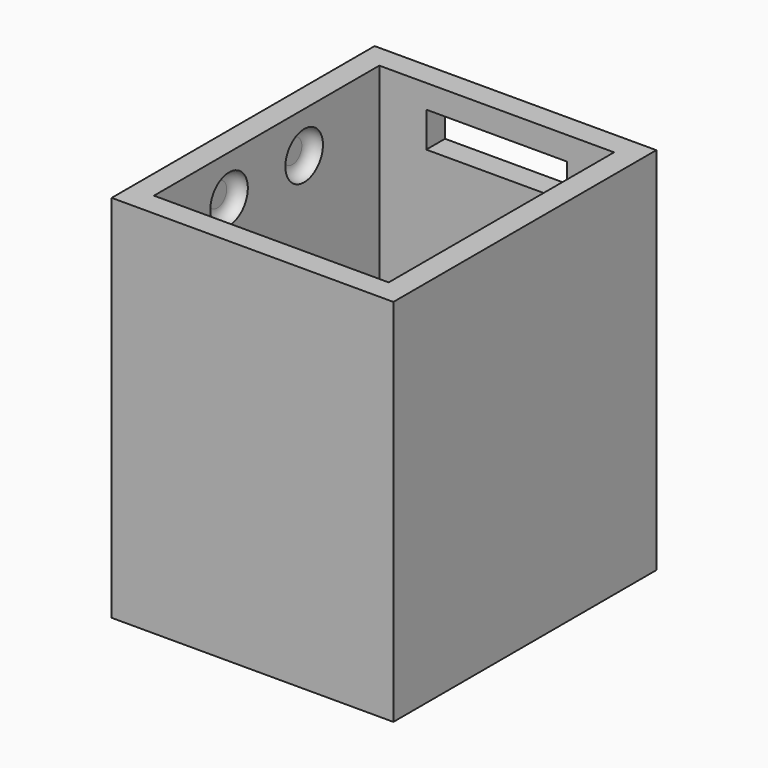
from build123d import *

# Parameters (mm, degrees)
F0_W      = 24
F0_H      = 28
F0_W_2    = 15
F0_H_2    = 20
F1_DEPTH  = 1.5
F2_W      = 24
F2_H      = 28
F2_W_2    = 20
F2_H_2    = 24
F3_DEPTH  = 30
F4_R      = 2
F5_DEPTH  = 1
F6_R      = 2
F7_DEPTH  = 1
F8_R      = 0.99999
F9_W      = 12
F9_H      = 3
F10_DEPTH = 2


# Not quite as in the source:
# - a fillet or chamfer is up to 0.001 mm smaller than in the source, because OpenCascade refuses the exact size


with BuildPart() as f1:
    # F0 (on Top) → F1 (new body)
    with BuildSketch(Plane.XY):
        Rectangle(F0_W, F0_H)
        Rectangle(F0_W_2, F0_H_2, mode=Mode.SUBTRACT)
    extrude(amount=F1_DEPTH)

    # F2 (on face) → F3 (join)
    with BuildSketch(Plane.XY.offset(1.5)):
        Rectangle(F2_W, F2_H)
        Rectangle(F2_W_2, F2_H_2, mode=Mode.SUBTRACT)
    extrude(amount=F3_DEPTH)

    # F4 (on face) → F5 (cut)
    with BuildSketch(Plane.YZ.offset(-10)):
        with Locations((-4, 28)):
            Circle(F4_R)
        with Locations((4, 28)):
            Circle(F4_R)
    extrude(amount=-F5_DEPTH, mode=Mode.SUBTRACT)

    # F6 (on face) → F7 (cut)
    with BuildSketch(Plane(origin=(10, 0, 0), x_dir=(0, -1, 0), z_dir=(-1, 0, 0))):
        with Locations((4, 28)):
            Circle(F6_R)
        with Locations((-4, 28)):
            Circle(F6_R)
    extrude(amount=-F7_DEPTH, mode=Mode.SUBTRACT)

    # F8 (radius 1 in the source; OpenCascade refuses exactly that, so slightly less here)
    f8_edges = [f1.edges().sort_by_distance(p)[0] for p in [
        (11, -2, 28),
        (11, 6, 28),
        (-11, -6, 28),
        (-11, 2, 28),
    ]]
    fillet(f8_edges, radius=F8_R)

    # F9 (on face) → F10 (cut, through all)
    with BuildSketch(Plane(origin=(0, 14, 0), x_dir=(-1, 0, 0), z_dir=(0, 1, 0))):
        with Locations((0, 28)):
            Rectangle(F9_W, F9_H)
    extrude(amount=-F10_DEPTH, mode=Mode.SUBTRACT)


solid = f1.part
